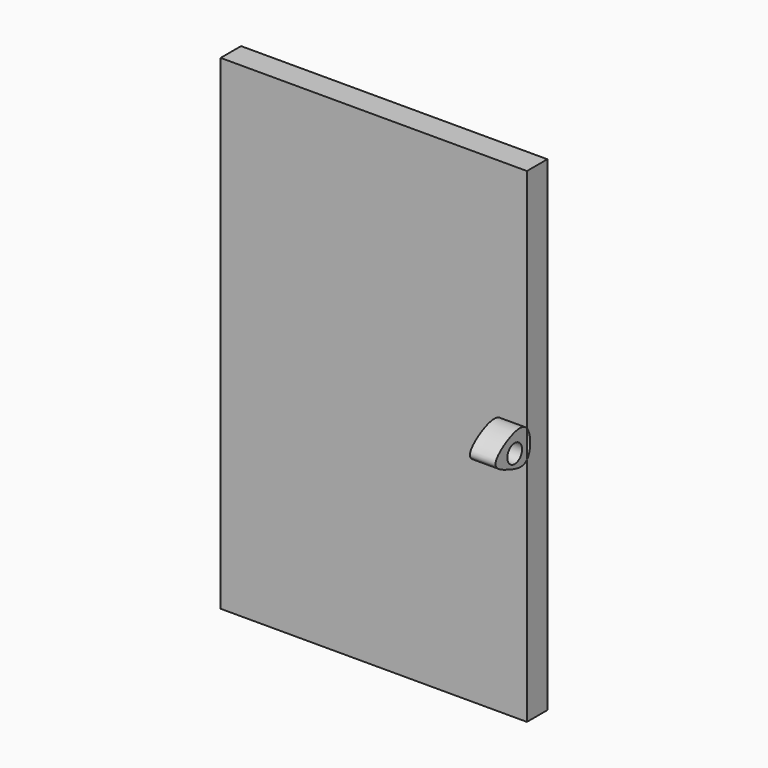
from build123d import *

# Parameters (mm, degrees)
F0_W     = 279.4
F0_H     = 482.6
F1_DEPTH = 25.4
F2_R     = 9.2101636832
F3_DEPTH = 25.4


with BuildPart() as f1:
    # F0 (on Front) → F1 (new body)
    with BuildSketch(Plane.XZ):
        Rectangle(F0_W, F0_H)
    extrude(amount=F1_DEPTH)

    # F2 (on face) → F3 (join)
    with BuildSketch(Plane.YZ.offset(139.7)):
        with BuildLine():
            Line((-25.4, -11.7313759401), (-25.4, 15.8898923546))
            add(Edge.make_bspline(
                [(-25.4, 15.8898923546), (-30.2232915007, 21.6659738224), (-48.5578217968, 18.3532526749), (-72.3516137088, -1.0281140256), (-48.6982925667, -11.4593535624), (-30.3847897858, -17.051569857), (-25.4, -11.7313759401)],
                knots=[0, 0, 0, 0, 0.1979250123, 0.3974815266, 0.5791241072, 0.7811204339, 0.7811204339, 0.7811204339, 0.7811204339], degree=3))
        make_face()
        with Locations((-40.6200774014, 0)):
            Circle(F2_R, mode=Mode.SUBTRACT)
        with BuildLine():
            Line((-25.4, 241.3), (-25.4, 15.8898923546))
            add(Edge.make_bspline(
                [(-25.4, -11.7313759401), (-19.9985719489, -5.9665100391), (-20.0660609566, 9.5022903499), (-25.4, 15.8898923546)],
                knots=[0.7811204339, 0.7811204339, 0.7811204339, 0.7811204339, 1, 1, 1, 1], degree=3))
            Line((-25.4, -11.7313759401), (-25.4, -241.3))
            Line((-25.4, -241.3), (0, -241.3))
            Line((0, -241.3), (0, 241.3))
            Line((0, 241.3), (-25.4, 241.3))
        make_face()
    extrude(amount=F3_DEPTH)


solid = f1.part
